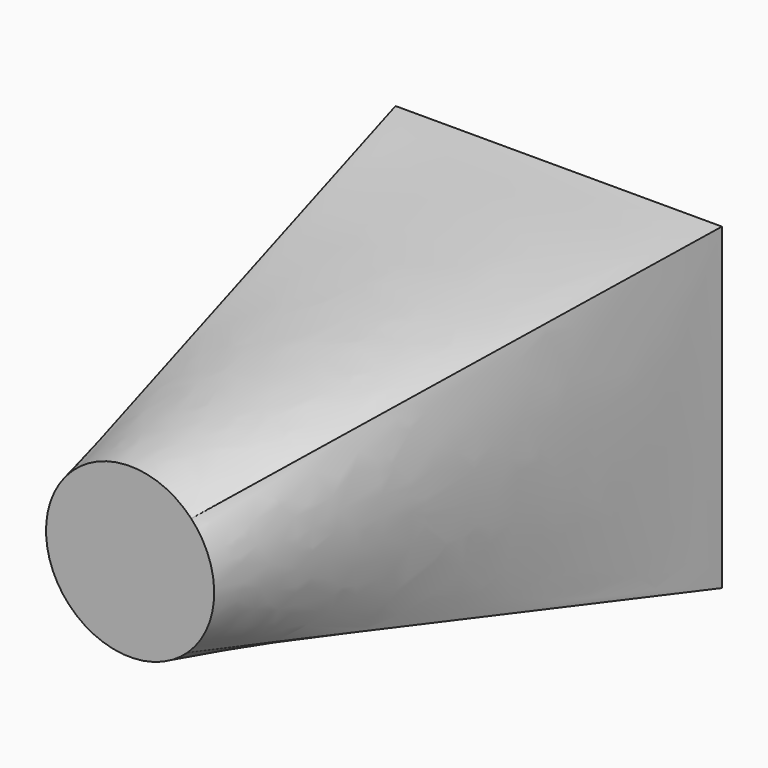
from build123d import *

# Parameters (mm, degrees)
F0_W = 65.3142854571
F0_H = 63.6814311147


# Not quite as in the source:
# - the arcs of a loft's sections are written as splines that run evenly, so that the points pair up as in the source's solid


with BuildPart() as f3:
    # F0 (on Front) → F3 section 0
    with BuildSketch(Plane.XZ):
        with Locations((4.4903568923, -2.0410716534)):
            Rectangle(F0_W, F0_H)
    # F2 (on offset) → F3 section 1
    with BuildSketch(Plane.XZ.offset(101.6)):
        with BuildLine():
            add(Edge.make_bspline(
                [(-11.5590845015, 12.2291767334), (-12.3594822471, 11.4726364219), (-13.0853493267, 10.6372844694), (-14.3601985952, 8.8409775584), (-14.909149261, 7.8800670172), (-15.8090605647, 5.8695648855), (-16.1599989505, 4.8200230087), (-16.6503892025, 2.6725881258), (-16.7898289428, 1.5747482191), (-16.8518527208, -0.6270946969), (-16.7744352248, -1.7310432614), (-16.4057089898, -3.902678622), (-16.1144093683, -4.9703117201), (-15.3291030627, -7.0282847963), (-14.8351157968, -8.0185738869), (-13.6634083015, -9.8837979274), (-12.9857170449, -10.758686756), (-12.2291767334, -11.5590845015)],
                knots=[0, 0, 0, 0, 0.125, 0.125, 0.25, 0.25, 0.375, 0.375, 0.5, 0.5, 0.625, 0.625, 0.75, 0.75, 0.875, 0.875, 1, 1, 1, 1], degree=3))
            add(Edge.make_bspline(
                [(-12.2291767334, -11.5590845015), (-11.4726364219, -12.3594822471), (-10.6372844694, -13.0853493267), (-8.8409775584, -14.3601985952), (-7.8800670172, -14.909149261), (-5.8695648855, -15.8090605647), (-4.8200230087, -16.1599989505), (-2.6725881258, -16.6503892025), (-1.5747482191, -16.7898289428), (0.6270946969, -16.8518527208), (1.7310432614, -16.7744352248), (3.902678622, -16.4057089898), (4.9703117201, -16.1144093683), (7.0282847963, -15.3291030627), (8.0185738869, -14.8351157968), (9.8837979274, -13.6634083015), (10.758686756, -12.9857170449), (11.5590845015, -12.2291767334)],
                knots=[0, 0, 0, 0, 0.125, 0.125, 0.25, 0.25, 0.375, 0.375, 0.5, 0.5, 0.625, 0.625, 0.75, 0.75, 0.875, 0.875, 1, 1, 1, 1], degree=3))
            add(Edge.make_bspline(
                [(11.5590845015, -12.2291767334), (12.3594822471, -11.4726364219), (13.0853493267, -10.6372844694), (14.3601985952, -8.8409775584), (14.909149261, -7.8800670172), (15.8090605647, -5.8695648855), (16.1599989505, -4.8200230087), (16.6503892025, -2.6725881258), (16.7898289428, -1.5747482191), (16.8518527208, 0.6270946969), (16.7744352248, 1.7310432614), (16.4057089898, 3.902678622), (16.1144093683, 4.9703117201), (15.3291030627, 7.0282847963), (14.8351157968, 8.0185738869), (13.6634083015, 9.8837979274), (12.9857170449, 10.758686756), (12.2291767334, 11.5590845015)],
                knots=[0, 0, 0, 0, 0.125, 0.125, 0.25, 0.25, 0.375, 0.375, 0.5, 0.5, 0.625, 0.625, 0.75, 0.75, 0.875, 0.875, 1, 1, 1, 1], degree=3))
            add(Edge.make_bspline(
                [(12.2291767334, 11.5590845015), (11.4726364219, 12.3594822471), (10.6372844694, 13.0853493267), (8.8409775584, 14.3601985952), (7.8800670172, 14.909149261), (5.8695648855, 15.8090605647), (4.8200230087, 16.1599989505), (2.6725881258, 16.6503892025), (1.5747482191, 16.7898289428), (-0.6270946969, 16.8518527208), (-1.7310432614, 16.7744352248), (-3.902678622, 16.4057089898), (-4.9703117201, 16.1144093683), (-7.0282847963, 15.3291030627), (-8.0185738869, 14.8351157968), (-9.8837979274, 13.6634083015), (-10.758686756, 12.9857170449), (-11.5590845015, 12.2291767334)],
                knots=[0, 0, 0, 0, 0.125, 0.125, 0.25, 0.25, 0.375, 0.375, 0.5, 0.5, 0.625, 0.625, 0.75, 0.75, 0.875, 0.875, 1, 1, 1, 1], degree=3))
        make_face()
    loft(ruled=True)


solid = f3.part
